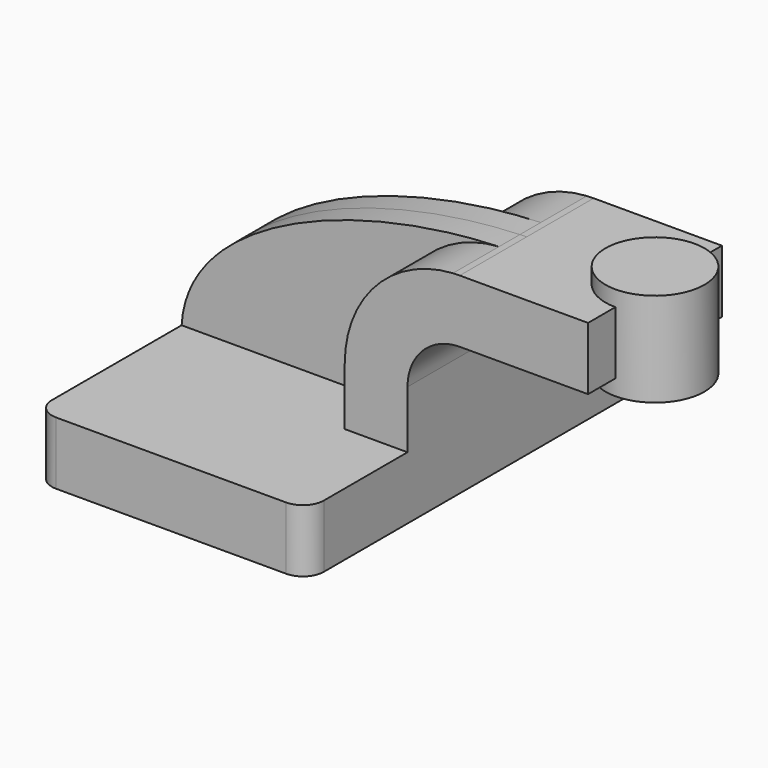
from build123d import *

# Parameters (mm, degrees)
F1_DEPTH = 63.5
F0_W     = 35.7702043533
F0_H     = 19.0499988828
F2_DEPTH = 25.4
F3_DEPTH = 7.9375
F5_R     = 6.35


# Not quite as in the source:
# - ends of sketch curves that miss each other by under 0.0002 mm in the source are joined


with BuildPart() as f1:
    # F0 (on Front) → F1 (new body, symmetric)
    with BuildSketch(Plane.XZ):
        Polygon((-41.275, -9.525), (41.275, -9.525), (41.275, 9.525), (22.225, 9.525), (-41.275, 9.525), align=None)
    extrude(amount=F1_DEPTH, both=True)

    # F0 (on Front) → F2 (join, symmetric)
    with BuildSketch(Plane.XZ):
        with BuildLine():
            Line((22.225, 9.525), (41.275, 9.525))
            Line((41.275, 9.525), (41.275, 27.0002))
            ThreePointArc((41.275, 27.0002), (45.9246798487, 38.2255201513), (57.15, 42.8752))
            Line((57.15, 42.8752), (60.325, 42.8752))
            Line((60.325, 42.8752), (60.325, 61.9251988828))
            Line((60.325, 61.9251988828), (57.15, 61.9251988828))
            add(Edge.make_bspline(
                [(55.0732880095, 61.8634025538), (55.7666834516, 61.8883145564), (56.4589847756, 61.9089220973), (57.15, 61.9251988828)],
                knots=[109.8121329902, 109.8121329902, 109.8121329902, 109.8121329902, 111.5045361635, 111.5045361635, 111.5045361635, 111.5045361635], degree=3))
            ThreePointArc((55.0732880095, 61.8634025538), (31.7306688594, 50.9504239941), (22.225, 27.0002))
            Line((22.225, 27.0002), (22.225, 9.525))
        make_face()
        with Locations((78.2101021767, 52.4001994414)):
            Rectangle(F0_W, F0_H)
    extrude(amount=F2_DEPTH, both=True)

    # F0 (on Front) → F3 (join, symmetric)
    with BuildSketch(Plane.XZ):
        with BuildLine():
            add(Edge.make_bspline(
                [(-41.275, 9.525), (-39.5154446815, 40.5083175564), (10.0820981423, 60.2469791277), (55.0732880095, 61.8634025538)],
                knots=[0, 0, 0, 0, 109.8121329902, 109.8121329902, 109.8121329902, 109.8121329902], degree=3))
            Line((-41.275, 9.525), (22.225, 9.525))
            Line((22.225, 9.525), (22.225, 27.0002))
            ThreePointArc((22.225, 27.0002), (31.7306688594, 50.9504239941), (55.0732880095, 61.8634025538))
        make_face()
    extrude(amount=F3_DEPTH, both=True)

    # F0 (on Front) → F4 (revolve)
    with BuildSketch(Plane.XZ):
        Polygon((96.0952043533, 61.9251988828), (96.0952043533, 42.8752), (96.0952043533, 38.1), (111.125, 38.1), (111.125, 66.675), (96.0952043533, 66.675), align=None)
    revolve(axis=Axis((96.0952043533, 0, 52.3875), (0, 0, -1)))

    # F5
    f5_edges = [f1.edges().sort_by_distance(p)[0] for p in [
        (41.275, -63.5, 0),
        (-41.275, -63.5, 0),
        (41.275, 63.5, 0),
        (-41.275, 63.5, 0),
    ]]
    fillet(f5_edges, radius=F5_R)


solid = f1.part
